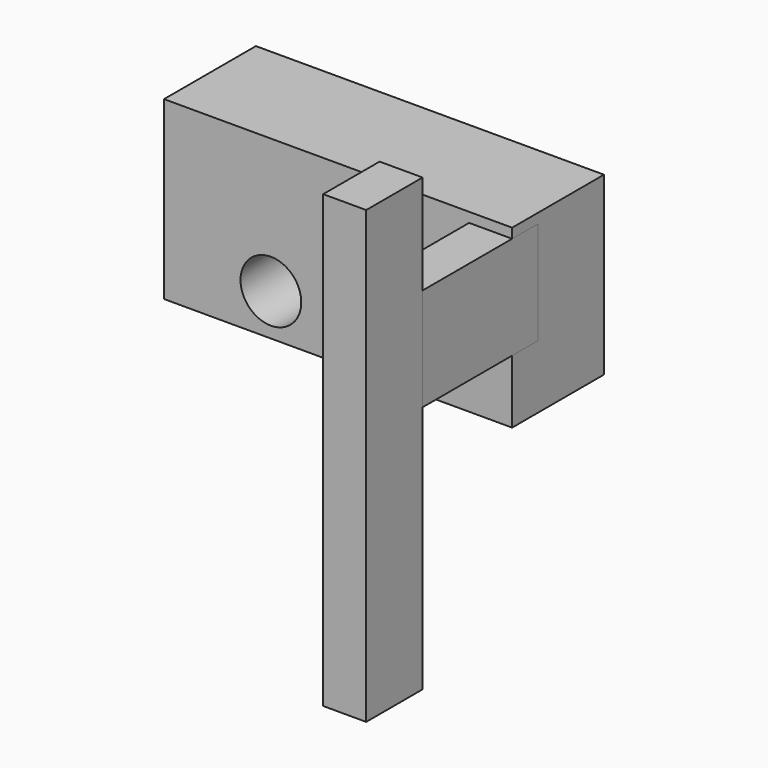
from build123d import *

# Parameters (mm, degrees)
F0_W     = 12.1247209609
F0_H     = 19.86515522
F2_DEPTH = 127
F3_W     = 32.3565304279
F3_H     = 49.6104732156
F4_DEPTH = 98.0996470898
F6_W     = 12.1247209609
F6_H     = 28.984606266
F7_DEPTH = 40.7187305391
F8_R     = 8.5562099795
F9_DEPTH = 81.7973520607


# Not quite as in the source:
# - a feature of the source that left no trace in its solid (it failed there, or was rolled back) is left out


with BuildPart() as f2:
    # F0 (on Top) → F2 (new body)
    with BuildSketch(Plane.XY):
        with Locations((45.3508067876, -41.4686575532)):
            Rectangle(F0_W, F0_H)
    extrude(amount=F2_DEPTH)


with BuildPart() as f4:
    # F3 (on face) → F4 (new body)
    with BuildSketch(Plane.YZ.offset(51.413167268)):
        with Locations((16.178265214, 76.9235752523)):
            Rectangle(F3_W, F3_H)
    extrude(amount=-F4_DEPTH)

    # F8 (on face) → F9 (cut)
    with BuildSketch(Plane(origin=(0, 32.3565304279, 0), x_dir=(-1, 0, 0), z_dir=(0, 1, 0))):
        with Locations((16.5728703141, 63.8606324792)):
            Circle(F8_R)
    extrude(amount=-F9_DEPTH, mode=Mode.SUBTRACT)


with BuildPart() as f7:
    # F6 (on face) → F7 (new body)
    with BuildSketch(Plane(origin=(0, -31.5360799432, 0), x_dir=(-1, 0, 0), z_dir=(0, 1, 0))):
        with Locations((-45.3508067876, 84.4837799668)):
            Rectangle(F6_W, F6_H)
    extrude(amount=F7_DEPTH)


solid = Compound([f2.part, f4.part, f7.part])
